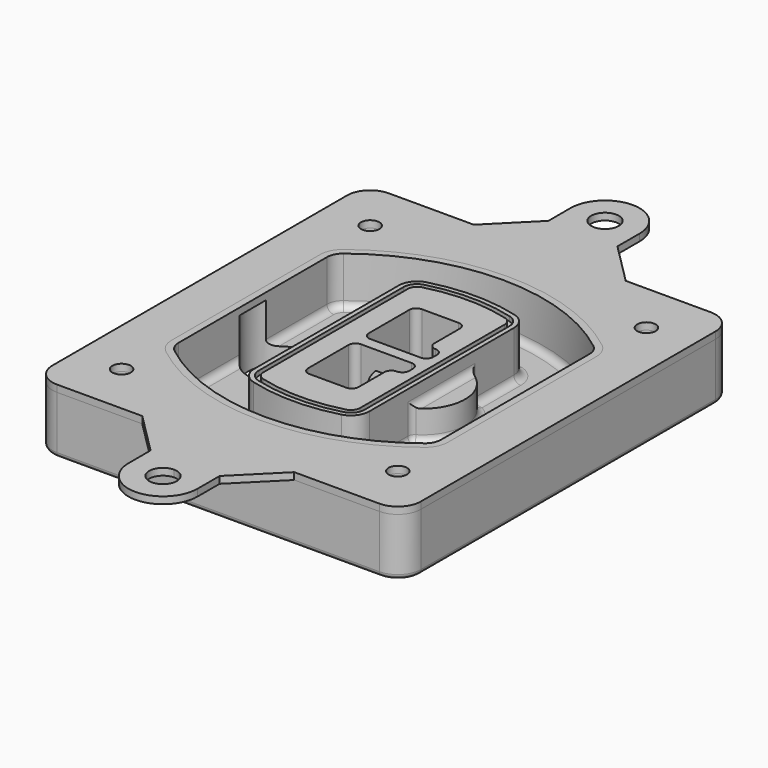
from build123d import *

# Parameters (mm, degrees)
F0_R      = 4
F1_DEPTH  = 25
F2_DEPTH  = 3
F3_DEPTH  = 18
F5_DEPTH  = 21
F6_DEPTH  = 2
F8_DEPTH  = 20
F9_DEPTH  = 16
F10_DEPTH = 25
F7_R      = 6
F7_R_2    = 4
F11_DEPTH = 6
F13_DEPTH = 9
F14_R     = 3
F15_R     = 2
F16_R     = 4
F17_DEPTH = 3


with BuildPart() as f1:
    # F0 (on Top) → F1 (new body)
    with BuildSketch(Plane.XY):
        with BuildLine():
            ThreePointArc((-80, -80), (-77.0710678119, -87.0710678119), (-70, -90))
            Line((-70, -90), (70, -90))
            ThreePointArc((70, -90), (77.0710678119, -87.0710678119), (80, -80))
            Line((80, -80), (80, 80))
            ThreePointArc((80, 80), (77.0710678119, 87.0710678119), (70, 90))
            Line((70, 90), (-70, 90))
            ThreePointArc((-70, 90), (-77.0710678119, 87.0710678119), (-80, 80))
            Line((-80, 80), (-80, -80))
        make_face()
        with Locations((-60, -67.5)):
            Circle(F0_R, mode=Mode.SUBTRACT)
        with Locations((60, -67.5)):
            Circle(F0_R, mode=Mode.SUBTRACT)
        with Locations((-60, 67.5)):
            Circle(F0_R, mode=Mode.SUBTRACT)
        with BuildLine():
            ThreePointArc((-64, 40.2934422872), (-62.5820384798, 46.4328484224), (-58.6153846154, 51.3286200352))
            ThreePointArc((-58.6153846154, 51.3286200352), (0, 71.5), (58.6153846154, 51.3286200352))
            ThreePointArc((58.6153846154, 51.3286200352), (62.5820384798, 46.4328484224), (64, 40.2934422872))
            Line((64, 40.2934422872), (64, -40.2934422872))
            ThreePointArc((64, -40.2934422872), (62.5820384798, -46.4328484224), (58.6153846154, -51.3286200352))
            ThreePointArc((58.6153846154, -51.3286200352), (0, -71.5), (-58.6153846154, -51.3286200352))
            ThreePointArc((-58.6153846154, -51.3286200352), (-62.5820384798, -46.4328484224), (-64, -40.2934422872))
            Line((-64, -40.2934422872), (-64, 40.2934422872))
        make_face(mode=Mode.SUBTRACT)
        with Locations((60, 67.5)):
            Circle(F0_R, mode=Mode.SUBTRACT)
        with BuildLine():
            ThreePointArc((58.6153846154, 51.3286200352), (0, 71.5), (-58.6153846154, 51.3286200352))
            ThreePointArc((-58.6153846154, 51.3286200352), (-62.5820384798, 46.4328484224), (-64, 40.2934422872))
            Line((-64, 40.2934422872), (-64, -40.2934422872))
            ThreePointArc((-64, -40.2934422872), (-62.5820384798, -46.4328484224), (-58.6153846154, -51.3286200352))
            ThreePointArc((-58.6153846154, -51.3286200352), (0, -71.5), (58.6153846154, -51.3286200352))
            ThreePointArc((58.6153846154, -51.3286200352), (62.5820384798, -46.4328484224), (64, -40.2934422872))
            Line((64, -40.2934422872), (64, 40.2934422872))
            ThreePointArc((64, 40.2934422872), (62.5820384798, 46.4328484224), (58.6153846154, 51.3286200352))
        make_face()
        with BuildLine():
            Line((-60, -40.2934422872), (-60, 40.2934422872))
            ThreePointArc((-60, 40.2934422872), (-58.9871703427, 44.6787323838), (-56.1538461538, 48.1757121072))
            ThreePointArc((-56.1538461538, 48.1757121072), (0, 67.5), (56.1538461538, 48.1757121072))
            ThreePointArc((56.1538461538, 48.1757121072), (58.9871703427, 44.6787323838), (60, 40.2934422872))
            Line((60, 40.2934422872), (60, -40.2934422872))
            ThreePointArc((60, -40.2934422872), (58.9871703427, -44.6787323838), (56.1538461538, -48.1757121072))
            ThreePointArc((56.1538461538, -48.1757121072), (0, -67.5), (-56.1538461538, -48.1757121072))
            ThreePointArc((-56.1538461538, -48.1757121072), (-58.9871703427, -44.6787323838), (-60, -40.2934422872))
        make_face(mode=Mode.SUBTRACT)
        with BuildLine():
            ThreePointArc((-56.1538461538, 48.1757121072), (-58.9871703427, 44.6787323838), (-60, 40.2934422872))
            Line((-60, 40.2934422872), (-60, -40.2934422872))
            ThreePointArc((-60, -40.2934422872), (-58.9871703427, -44.6787323838), (-56.1538461538, -48.1757121072))
            ThreePointArc((-56.1538461538, -48.1757121072), (0, -67.5), (56.1538461538, -48.1757121072))
            ThreePointArc((56.1538461538, -48.1757121072), (58.9871703427, -44.6787323838), (60, -40.2934422872))
            Line((60, -40.2934422872), (60, 40.2934422872))
            ThreePointArc((60, 40.2934422872), (58.9871703427, 44.6787323838), (56.1538461538, 48.1757121072))
            ThreePointArc((56.1538461538, 48.1757121072), (0, 67.5), (-56.1538461538, 48.1757121072))
        make_face()
        with BuildLine():
            ThreePointArc((54.3076923077, 45.8110311612), (56.2910192399, 43.3631453548), (57, 40.2934422872))
            Line((57, 40.2934422872), (57, -40.2934422872))
            ThreePointArc((57, -40.2934422872), (56.2910192399, -43.3631453548), (54.3076923077, -45.8110311612))
            ThreePointArc((54.3076923077, -45.8110311612), (0, -64.5), (-54.3076923077, -45.8110311612))
            ThreePointArc((-54.3076923077, -45.8110311612), (-56.2910192399, -43.3631453548), (-57, -40.2934422872))
            Line((-57, -40.2934422872), (-57, 40.2934422872))
            ThreePointArc((-57, 40.2934422872), (-56.2910192399, 43.3631453548), (-54.3076923077, 45.8110311612))
            ThreePointArc((-54.3076923077, 45.8110311612), (0, 64.5), (54.3076923077, 45.8110311612))
        make_face(mode=Mode.SUBTRACT)
        with BuildLine():
            Line((57, -40.2934422872), (57, 40.2934422872))
            ThreePointArc((57, 40.2934422872), (56.2910192399, 43.3631453548), (54.3076923077, 45.8110311612))
            ThreePointArc((54.3076923077, 45.8110311612), (0, 64.5), (-54.3076923077, 45.8110311612))
            ThreePointArc((-54.3076923077, 45.8110311612), (-56.2910192399, 43.3631453548), (-57, 40.2934422872))
            Line((-57, 40.2934422872), (-57, -40.2934422872))
            ThreePointArc((-57, -40.2934422872), (-56.2910192399, -43.3631453548), (-54.3076923077, -45.8110311612))
            ThreePointArc((-54.3076923077, -45.8110311612), (0, -64.5), (54.3076923077, -45.8110311612))
            ThreePointArc((54.3076923077, -45.8110311612), (56.2910192399, -43.3631453548), (57, -40.2934422872))
        make_face()
    extrude(amount=-F1_DEPTH)

    # F0 (on Top) → F2 (join)
    with BuildSketch(Plane.XY):
        with BuildLine():
            ThreePointArc((-56.1538461538, 48.1757121072), (-58.9871703427, 44.6787323838), (-60, 40.2934422872))
            Line((-60, 40.2934422872), (-60, -40.2934422872))
            ThreePointArc((-60, -40.2934422872), (-58.9871703427, -44.6787323838), (-56.1538461538, -48.1757121072))
            ThreePointArc((-56.1538461538, -48.1757121072), (0, -67.5), (56.1538461538, -48.1757121072))
            ThreePointArc((56.1538461538, -48.1757121072), (58.9871703427, -44.6787323838), (60, -40.2934422872))
            Line((60, -40.2934422872), (60, 40.2934422872))
            ThreePointArc((60, 40.2934422872), (58.9871703427, 44.6787323838), (56.1538461538, 48.1757121072))
            ThreePointArc((56.1538461538, 48.1757121072), (0, 67.5), (-56.1538461538, 48.1757121072))
        make_face()
        with BuildLine():
            ThreePointArc((54.3076923077, 45.8110311612), (56.2910192399, 43.3631453548), (57, 40.2934422872))
            Line((57, 40.2934422872), (57, -40.2934422872))
            ThreePointArc((57, -40.2934422872), (56.2910192399, -43.3631453548), (54.3076923077, -45.8110311612))
            ThreePointArc((54.3076923077, -45.8110311612), (0, -64.5), (-54.3076923077, -45.8110311612))
            ThreePointArc((-54.3076923077, -45.8110311612), (-56.2910192399, -43.3631453548), (-57, -40.2934422872))
            Line((-57, -40.2934422872), (-57, 40.2934422872))
            ThreePointArc((-57, 40.2934422872), (-56.2910192399, 43.3631453548), (-54.3076923077, 45.8110311612))
            ThreePointArc((-54.3076923077, 45.8110311612), (0, 64.5), (54.3076923077, 45.8110311612))
        make_face(mode=Mode.SUBTRACT)
    extrude(amount=F2_DEPTH)

    # F0 (on Top) → F3 (cut)
    with BuildSketch(Plane.XY):
        with BuildLine():
            Line((57, -40.2934422872), (57, 40.2934422872))
            ThreePointArc((57, 40.2934422872), (56.2910192399, 43.3631453548), (54.3076923077, 45.8110311612))
            ThreePointArc((54.3076923077, 45.8110311612), (0, 64.5), (-54.3076923077, 45.8110311612))
            ThreePointArc((-54.3076923077, 45.8110311612), (-56.2910192399, 43.3631453548), (-57, 40.2934422872))
            Line((-57, 40.2934422872), (-57, -40.2934422872))
            ThreePointArc((-57, -40.2934422872), (-56.2910192399, -43.3631453548), (-54.3076923077, -45.8110311612))
            ThreePointArc((-54.3076923077, -45.8110311612), (0, -64.5), (54.3076923077, -45.8110311612))
            ThreePointArc((54.3076923077, -45.8110311612), (56.2910192399, -43.3631453548), (57, -40.2934422872))
        make_face()
    extrude(amount=-F3_DEPTH, mode=Mode.SUBTRACT)

    # F4 (on face) → F5 (join, through all)
    with BuildSketch(Plane.XY.offset(3)):
        with BuildLine():
            ThreePointArc((-25, -39.2465276821), (-23.3511545998, -44.1109737193), (-19.0842911877, -46.9702398883))
            ThreePointArc((-19.0842911877, -46.9702398883), (0, -49.5), (19.0842911877, -46.9702398883))
            ThreePointArc((19.0842911877, -46.9702398883), (23.3511545998, -44.1109737193), (25, -39.2465276821))
            Line((25, -39.2465276821), (25, 39.2465276821))
            ThreePointArc((25, 39.2465276821), (23.3511545998, 44.1109737193), (19.0842911877, 46.9702398883))
            ThreePointArc((19.0842911877, 46.9702398883), (0, 49.5), (-19.0842911877, 46.9702398883))
            ThreePointArc((-19.0842911877, 46.9702398883), (-23.3511545998, 44.1109737193), (-25, 39.2465276821))
            Line((-25, 39.2465276821), (-25, -39.2465276821))
        make_face()
        with BuildLine():
            ThreePointArc((18.5632183908, 45.0393118368), (21.7633659499, 42.89486221), (23, 39.2465276821))
            Line((23, 39.2465276821), (23, -39.2465276821))
            ThreePointArc((23, -39.2465276821), (21.7633659499, -42.89486221), (18.5632183908, -45.0393118368))
            ThreePointArc((18.5632183908, -45.0393118368), (0, -47.5), (-18.5632183908, -45.0393118368))
            ThreePointArc((-18.5632183908, -45.0393118368), (-21.7633659499, -42.89486221), (-23, -39.2465276821))
            Line((-23, -39.2465276821), (-23, 39.2465276821))
            ThreePointArc((-23, 39.2465276821), (-21.7633659499, 42.89486221), (-18.5632183908, 45.0393118368))
            ThreePointArc((-18.5632183908, 45.0393118368), (0, 47.5), (18.5632183908, 45.0393118368))
        make_face(mode=Mode.SUBTRACT)
        with BuildLine():
            Line((23, -39.2465276821), (23, 39.2465276821))
            ThreePointArc((23, 39.2465276821), (21.7633659499, 42.89486221), (18.5632183908, 45.0393118368))
            ThreePointArc((18.5632183908, 45.0393118368), (0, 47.5), (-18.5632183908, 45.0393118368))
            ThreePointArc((-18.5632183908, 45.0393118368), (-21.7633659499, 42.89486221), (-23, 39.2465276821))
            Line((-23, 39.2465276821), (-23, -39.2465276821))
            ThreePointArc((-23, -39.2465276821), (-21.7633659499, -42.89486221), (-18.5632183908, -45.0393118368))
            ThreePointArc((-18.5632183908, -45.0393118368), (0, -47.5), (18.5632183908, -45.0393118368))
            ThreePointArc((18.5632183908, -45.0393118368), (21.7633659499, -42.89486221), (23, -39.2465276821))
        make_face()
        with BuildLine():
            ThreePointArc((18.0421455939, 43.1083837852), (20.1755772999, 41.6787507007), (21, 39.2465276821))
            Line((21, 39.2465276821), (21, -39.2465276821))
            ThreePointArc((21, -39.2465276821), (20.1755772999, -41.6787507007), (18.0421455939, -43.1083837852))
            ThreePointArc((18.0421455939, -43.1083837852), (0, -45.5), (-18.0421455939, -43.1083837852))
            ThreePointArc((-18.0421455939, -43.1083837852), (-20.1755772999, -41.6787507007), (-21, -39.2465276821))
            Line((-21, -39.2465276821), (-21, 39.2465276821))
            ThreePointArc((-21, 39.2465276821), (-20.1755772999, 41.6787507007), (-18.0421455939, 43.1083837852))
            ThreePointArc((-18.0421455939, 43.1083837852), (0, 45.5), (18.0421455939, 43.1083837852))
        make_face(mode=Mode.SUBTRACT)
        with BuildLine():
            Line((21, -39.2465276821), (21, 39.2465276821))
            ThreePointArc((21, 39.2465276821), (20.1755772999, 41.6787507007), (18.0421455939, 43.1083837852))
            ThreePointArc((18.0421455939, 43.1083837852), (0, 45.5), (-18.0421455939, 43.1083837852))
            ThreePointArc((-18.0421455939, 43.1083837852), (-20.1755772999, 41.6787507007), (-21, 39.2465276821))
            Line((-21, 39.2465276821), (-21, -39.2465276821))
            ThreePointArc((-21, -39.2465276821), (-20.1755772999, -41.6787507007), (-18.0421455939, -43.1083837852))
            ThreePointArc((-18.0421455939, -43.1083837852), (0, -45.5), (18.0421455939, -43.1083837852))
            ThreePointArc((18.0421455939, -43.1083837852), (20.1755772999, -41.6787507007), (21, -39.2465276821))
        make_face()
        with BuildLine():
            Line((-8, -2.5), (14, -2.5))
            ThreePointArc((14, -2.5), (16.1213203436, -3.3786796564), (17, -5.5))
            Line((17, -5.5), (17, -7.5))
            ThreePointArc((17, -7.5), (16.1213203436, -9.6213203436), (14, -10.5))
            ThreePointArc((14, -10.5), (11.8786796564, -11.3786796564), (11, -13.5))
            Line((11, -13.5), (11, -27.5))
            ThreePointArc((11, -27.5), (10.1213203436, -29.6213203436), (8, -30.5))
            Line((8, -30.5), (-8, -30.5))
            ThreePointArc((-8, -30.5), (-10.1213203436, -29.6213203436), (-11, -27.5))
            Line((-11, -27.5), (-11, -5.5))
            ThreePointArc((-11, -5.5), (-10.1213203436, -3.3786796564), (-8, -2.5))
        make_face(mode=Mode.SUBTRACT)
        with BuildLine():
            ThreePointArc((-8, 2.5), (-10.1213203436, 3.3786796564), (-11, 5.5))
            Line((-11, 5.5), (-11, 27.5))
            ThreePointArc((-11, 27.5), (-10.1213203436, 29.6213203436), (-8, 30.5))
            Line((-8, 30.5), (8, 30.5))
            ThreePointArc((8, 30.5), (10.1213203436, 29.6213203436), (11, 27.5))
            Line((11, 27.5), (11, 13.5))
            ThreePointArc((11, 13.5), (11.8786796564, 11.3786796564), (14, 10.5))
            ThreePointArc((14, 10.5), (16.1213203436, 9.6213203436), (17, 7.5))
            Line((17, 7.5), (17, 5.5))
            ThreePointArc((17, 5.5), (16.1213203436, 3.3786796564), (14, 2.5))
            Line((14, 2.5), (-8, 2.5))
        make_face(mode=Mode.SUBTRACT)
    extrude(amount=-F5_DEPTH)

    # F4 (on face) → F6 (cut)
    with BuildSketch(Plane.XY.offset(3)):
        with BuildLine():
            Line((23, -39.2465276821), (23, 39.2465276821))
            ThreePointArc((23, 39.2465276821), (21.7633659499, 42.89486221), (18.5632183908, 45.0393118368))
            ThreePointArc((18.5632183908, 45.0393118368), (0, 47.5), (-18.5632183908, 45.0393118368))
            ThreePointArc((-18.5632183908, 45.0393118368), (-21.7633659499, 42.89486221), (-23, 39.2465276821))
            Line((-23, 39.2465276821), (-23, -39.2465276821))
            ThreePointArc((-23, -39.2465276821), (-21.7633659499, -42.89486221), (-18.5632183908, -45.0393118368))
            ThreePointArc((-18.5632183908, -45.0393118368), (0, -47.5), (18.5632183908, -45.0393118368))
            ThreePointArc((18.5632183908, -45.0393118368), (21.7633659499, -42.89486221), (23, -39.2465276821))
        make_face()
        with BuildLine():
            ThreePointArc((18.0421455939, 43.1083837852), (20.1755772999, 41.6787507007), (21, 39.2465276821))
            Line((21, 39.2465276821), (21, -39.2465276821))
            ThreePointArc((21, -39.2465276821), (20.1755772999, -41.6787507007), (18.0421455939, -43.1083837852))
            ThreePointArc((18.0421455939, -43.1083837852), (0, -45.5), (-18.0421455939, -43.1083837852))
            ThreePointArc((-18.0421455939, -43.1083837852), (-20.1755772999, -41.6787507007), (-21, -39.2465276821))
            Line((-21, -39.2465276821), (-21, 39.2465276821))
            ThreePointArc((-21, 39.2465276821), (-20.1755772999, 41.6787507007), (-18.0421455939, 43.1083837852))
            ThreePointArc((-18.0421455939, 43.1083837852), (0, 45.5), (18.0421455939, 43.1083837852))
        make_face(mode=Mode.SUBTRACT)
    extrude(amount=-F6_DEPTH, mode=Mode.SUBTRACT)

    # F7 (on face) → F8 (join)
    with BuildSketch(Plane(origin=(0, 0, -25), x_dir=(1, 0, 0), z_dir=(0, 0, -1))):
        with BuildLine():
            ThreePointArc((3.28842436, 0), (16.7567035675, 13.4682792075), (30.224982775, 0))
            Line((30.224982775, 0), (35.224982775, 0))
            ThreePointArc((35.224982775, 0), (16.7567035675, 18.4682792075), (-1.71157564, 0))
            Line((-1.71157564, 0), (3.28842436, 0))
        make_face()
        with BuildLine():
            Line((3.28842436, 0), (30.224982775, 0))
            ThreePointArc((30.224982775, 0), (16.7567035675, 13.4682792075), (3.28842436, 0))
        make_face()
        with BuildLine():
            ThreePointArc((3.28842436, 0), (16.7567035675, -13.4682792075), (30.224982775, 0))
            Line((30.224982775, 0), (3.28842436, 0))
        make_face()
        with BuildLine():
            Line((35.224982775, 0), (30.224982775, 0))
            ThreePointArc((30.224982775, 0), (16.7567035675, -13.4682792075), (3.28842436, 0))
            Line((3.28842436, 0), (-1.71157564, 0))
            ThreePointArc((-1.71157564, 0), (16.7567035675, -18.4682792075), (35.224982775, 0))
        make_face()
    extrude(amount=-F8_DEPTH)

    # F7 (on face) → F9 (cut)
    with BuildSketch(Plane(origin=(0, 0, -25), x_dir=(1, 0, 0), z_dir=(0, 0, -1))):
        with BuildLine():
            Line((3.28842436, 0), (30.224982775, 0))
            ThreePointArc((30.224982775, 0), (16.7567035675, 13.4682792075), (3.28842436, 0))
        make_face()
        with BuildLine():
            ThreePointArc((3.28842436, 0), (16.7567035675, -13.4682792075), (30.224982775, 0))
            Line((30.224982775, 0), (3.28842436, 0))
        make_face()
    extrude(amount=-F9_DEPTH, mode=Mode.SUBTRACT)

    # F7 (on face) → F10 (cut)
    with BuildSketch(Plane(origin=(0, 0, -25), x_dir=(1, 0, 0), z_dir=(0, 0, -1))):
        with BuildLine():
            Line((-59.0318229325, 0), (-32.0952645175, 0))
            ThreePointArc((-32.0952645175, 0), (-45.563543725, 13.4682792075), (-59.0318229325, 0))
        make_face()
        with BuildLine():
            ThreePointArc((-59.0318229325, 0), (-45.563543725, -13.4682792075), (-32.0952645175, 0))
            Line((-32.0952645175, 0), (-59.0318229325, 0))
        make_face()
    extrude(amount=-F10_DEPTH, mode=Mode.SUBTRACT)

    # F7 (on face) → F11 (cut)
    with BuildSketch(Plane(origin=(0, 0, -25), x_dir=(1, 0, 0), z_dir=(0, 0, -1))):
        with Locations((60, -67.5)):
            Circle(F7_R)
        with Locations((60, -67.5)):
            Circle(F7_R_2, mode=Mode.SUBTRACT)
        with Locations((-60, -67.5)):
            Circle(F7_R)
        with Locations((-60, -67.5)):
            Circle(F7_R_2, mode=Mode.SUBTRACT)
        with Locations((-60, 67.5)):
            Circle(F7_R)
        with Locations((-60, 67.5)):
            Circle(F7_R_2, mode=Mode.SUBTRACT)
        with Locations((60, 67.5)):
            Circle(F7_R)
        with Locations((60, 67.5)):
            Circle(F7_R_2, mode=Mode.SUBTRACT)
    extrude(amount=-F11_DEPTH, mode=Mode.SUBTRACT)

    # F12 (on face) → F13 (cut, through all)
    with BuildSketch(Plane(origin=(0, 0, -9), x_dir=(1, 0, 0), z_dir=(0, 0, -1))):
        with BuildLine():
            Line((11, 13.5), (11, 17.5481537753))
            ThreePointArc((11, 17.5481537753), (2.5696536419, 11.8239143813), (-1.5415842455, 2.5))
            Line((-1.5415842455, 2.5), (3.5224848595, 2.5))
            ThreePointArc((3.5224848595, 2.5), (6.1857188154, 8.3455872281), (11.2536447004, 12.2927168648))
            ThreePointArc((11.2536447004, 12.2927168648), (11.0640958889, 12.8831798879), (11, 13.5))
        make_face()
        with BuildLine():
            ThreePointArc((11.2536447004, -12.2927168648), (6.1857188154, -8.3455872281), (3.5224848595, -2.5))
            Line((3.5224848595, -2.5), (-1.5415842455, -2.5))
            ThreePointArc((-1.5415842455, -2.5), (2.5696536419, -11.8239143813), (11, -17.5481537753))
            Line((11, -17.5481537753), (11, -13.5))
            ThreePointArc((11, -13.5), (11.0640958889, -12.8831798879), (11.2536447004, -12.2927168648))
        make_face()
        with BuildLine():
            ThreePointArc((11.2536447004, 12.2927168648), (6.1857188154, 8.3455872281), (3.5224848595, 2.5))
            Line((3.5224848595, 2.5), (14, 2.5))
            ThreePointArc((14, 2.5), (16.1213203436, 3.3786796564), (17, 5.5))
            Line((17, 5.5), (17, 7.5))
            ThreePointArc((17, 7.5), (16.1213203436, 9.6213203436), (14, 10.5))
            ThreePointArc((14, 10.5), (12.3601599782, 10.9878446101), (11.2536447004, 12.2927168648))
        make_face()
        with BuildLine():
            Line((14, -2.5), (3.5224848595, -2.5))
            ThreePointArc((3.5224848595, -2.5), (6.1857188154, -8.3455872281), (11.2536447004, -12.2927168648))
            ThreePointArc((11.2536447004, -12.2927168648), (12.3601599782, -10.9878446101), (14, -10.5))
            ThreePointArc((14, -10.5), (16.1213203436, -9.6213203436), (17, -7.5))
            Line((17, -7.5), (17, -5.5))
            ThreePointArc((17, -5.5), (16.1213203436, -3.3786796564), (14, -2.5))
        make_face()
    extrude(amount=F13_DEPTH, mode=Mode.SUBTRACT)

    # F14
    f14_edges = [f1.edges().sort_by_distance(p)[0] for p in [
        (-57, -23.703476, -18),
        (-57, 23.703476, -18),
        (25, 0, -5),
        (25, 16.526506, -11.5),
        (25, -16.526506, -11.5),
        (25, -27.886517, -18),
        (35.224983, 0, -18),
    ]]
    fillet(f14_edges, radius=F14_R)

    # F15
    f15_edges = [f1.edges().sort_by_distance(p)[0] for p in [
        (0, -90, -25),
    ]]
    fillet(f15_edges, radius=F15_R)


with BuildPart() as f17:
    # F16 (on face) → F17 (new body, through all)
    with BuildSketch(Plane.XY):
        with BuildLine():
            Line((80, -80), (80, 0))
            Line((80, 0), (60, 0))
            Line((60, 0), (60, -40.2934422872))
            ThreePointArc((60, -40.2934422872), (58.9871703427, -44.6787323838), (56.1538461538, -48.1757121072))
            ThreePointArc((56.1538461538, -48.1757121072), (0, -67.5), (-56.1538461538, -48.1757121072))
            ThreePointArc((-56.1538461538, -48.1757121072), (-58.9871703427, -44.6787323838), (-60, -40.2934422872))
            Line((-60, -40.2934422872), (-60, 0))
            Line((-60, 0), (-80, 0))
            Line((-80, 0), (-80, -80))
            ThreePointArc((-80, -80), (-77.0710678119, -87.0710678119), (-70, -90))
            Line((-70, -90), (-33, -90))
            Line((-33, -90), (0, -90))
            Line((0, -90), (33, -90))
            Line((33, -90), (70, -90))
            ThreePointArc((70, -90), (77.0710678119, -87.0710678119), (80, -80))
        make_face()
        with Locations((-60, -67.5)):
            Circle(F16_R, mode=Mode.SUBTRACT)
        with Locations((60, -67.5)):
            Circle(F16_R, mode=Mode.SUBTRACT)
        with BuildLine():
            Line((15, -108), (33, -90))
            Line((33, -90), (0, -90))
            Line((0, -90), (-33, -90))
            Line((-33, -90), (-15, -108))
            Line((-15, -108), (-15, -120))
            ThreePointArc((-15, -120), (0, -135), (15, -120))
            Line((15, -120), (15, -108))
        make_face()
        with BuildLine():
            ThreePointArc((6, -120), (-4.2426406871, -124.2426406871), (0, -114))
            ThreePointArc((0, -114), (4.2426406871, -115.7573593129), (6, -120))
        make_face(mode=Mode.SUBTRACT)
        with BuildLine():
            Line((33, 90), (0, 90))
            Line((0, 90), (-33, 90))
            Line((-33, 90), (-70, 90))
            ThreePointArc((-70, 90), (-77.0710678119, 87.0710678119), (-80, 80))
            Line((-80, 80), (-80, 0))
            Line((-80, 0), (-60, 0))
            Line((-60, 0), (-60, 40.2934422872))
            ThreePointArc((-60, 40.2934422872), (-58.9871703427, 44.6787323838), (-56.1538461538, 48.1757121072))
            ThreePointArc((-56.1538461538, 48.1757121072), (0, 67.5), (56.1538461538, 48.1757121072))
            ThreePointArc((56.1538461538, 48.1757121072), (58.9871703427, 44.6787323838), (60, 40.2934422872))
            Line((60, 40.2934422872), (60, 0))
            Line((60, 0), (80, 0))
            Line((80, 0), (80, 80))
            ThreePointArc((80, 80), (77.0710678119, 87.0710678119), (70, 90))
            Line((70, 90), (33, 90))
        make_face()
        with Locations((-60, 67.5)):
            Circle(F16_R, mode=Mode.SUBTRACT)
        with Locations((60, 67.5)):
            Circle(F16_R, mode=Mode.SUBTRACT)
        with BuildLine():
            Line((-33, 90), (0, 90))
            Line((0, 90), (33, 90))
            Line((33, 90), (15, 108))
            Line((15, 108), (15, 120))
            ThreePointArc((15, 120), (0, 135), (-15, 120))
            Line((-15, 120), (-15, 108))
            Line((-15, 108), (-33, 90))
        make_face()
        with BuildLine():
            ThreePointArc((6, 120), (4.2426406871, 115.7573593129), (0, 114))
            ThreePointArc((0, 114), (-4.2426406871, 124.2426406871), (6, 120))
        make_face(mode=Mode.SUBTRACT)
    extrude(amount=F17_DEPTH)


solid = Compound([f1.part, f17.part])
